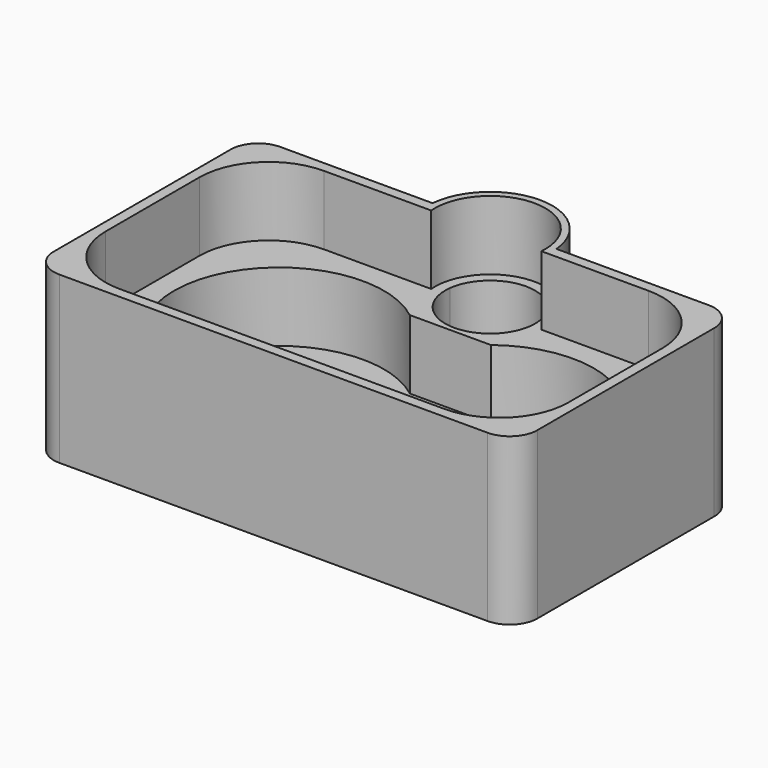
from build123d import *

# Parameters (mm, degrees)
F1_DEPTH = 2
F2_DEPTH = 5
F4_DEPTH = 5
F5_R     = 2
F6_R     = 5


# Not quite as in the source:
# - a feature names something its author has since deleted; it is built from what else it names


with BuildPart() as f1:
    # F0 (on Top) → F1 (new body)
    with BuildSketch(Plane.XY):
        with BuildLine():
            ThreePointArc((4.4821870069, 10), (0, 14.100000456), (-4.4821870069, 10))
            Line((-4.4821870069, 10), (-3.2252907411, 10))
            ThreePointArc((-3.2252907411, 10), (0, 12.850000456), (3.2252907411, 10))
            Line((3.2252907411, 10), (4.4821870069, 10))
        make_face()
        with BuildLine():
            Line((3.2252907411, 10), (-3.2252907411, 10))
            ThreePointArc((-3.2252907411, 10), (-0.2003810013, 6.3561836525), (3.25, 9.600000456))
            ThreePointArc((3.25, 9.600000456), (3.2438168034, 9.8003814573), (3.2252907411, 10))
        make_face()
        with BuildLine():
            ThreePointArc((3.2252907411, 10), (0, 12.850000456), (-3.2252907411, 10))
            Line((-3.2252907411, 10), (3.2252907411, 10))
        make_face()
        with BuildLine():
            ThreePointArc((-2.9352384841, 6), (-0.7731344117, 3.3397464334), (0, 0))
            ThreePointArc((0, 0), (0.7731344117, 3.3397464334), (2.9352384841, 6))
            Line((2.9352384841, 6), (2.699999392, 6))
            ThreePointArc((2.699999392, 6), (0, 5.100000456), (-2.699999392, 6))
            Line((-2.699999392, 6), (-2.9352384841, 6))
        make_face()
        with BuildLine():
            ThreePointArc((2.9352384841, -6), (0.7731344117, -3.3397464334), (0, 0))
            ThreePointArc((0, 0), (-0.7731344117, -3.3397464334), (-2.9352384841, -6))
            Line((-2.9352384841, -6), (2.9352384841, -6))
        make_face()
        with BuildLine():
            ThreePointArc((-4.4821870069, 10), (-4.1104683878, 7.768593993), (-2.699999392, 6))
            Line((-2.699999392, 6), (2.699999392, 6))
            ThreePointArc((2.699999392, 6), (4.0249221896, 7.5875389364), (4.5, 9.600000456))
            ThreePointArc((4.5, 9.600000456), (4.495544546, 9.8001984442), (4.4821870069, 10))
            Line((4.4821870069, 10), (3.2252907411, 10))
            ThreePointArc((3.2252907411, 10), (3.2438168034, 9.8003814573), (3.25, 9.600000456))
            ThreePointArc((3.25, 9.600000456), (-0.2003810013, 6.3561836525), (-3.2252907411, 10))
            Line((-3.2252907411, 10), (-4.4821870069, 10))
        make_face()
        with BuildLine():
            ThreePointArc((-2.9352384841, -6), (-0.7731344117, -3.3397464334), (0, 0))
            ThreePointArc((0, 0), (-0.7731344117, 3.3397464334), (-2.9352384841, 6))
            ThreePointArc((-2.9352384841, 6), (-14.6584577236, 2.8174766307), (-8.3490864524, -7.5629934211))
            ThreePointArc((-8.3490864524, -7.5629934211), (-7.6, -6.85), (-6.8509135476, -7.5629934211))
            ThreePointArc((-6.8509135476, -7.5629934211), (-4.7825233693, -7.0584577236), (-2.9352384841, -6))
        make_face()
        with BuildLine():
            ThreePointArc((2.9352384841, 6), (0.7731344117, 3.3397464334), (0, 0))
            ThreePointArc((0, 0), (0.7731344117, -3.3397464334), (2.9352384841, -6))
            ThreePointArc((2.9352384841, -6), (4.7825233693, -7.0584577236), (6.8509135476, -7.5629934211))
            ThreePointArc((6.8509135476, -7.5629934211), (7.6, -6.85), (8.3490864524, -7.5629934211))
            ThreePointArc((8.3490864524, -7.5629934211), (13.2326306926, -5.1023006067), (15.2, 0))
            ThreePointArc((15.2, 0), (10.9397464334, 6.8268655883), (2.9352384841, 6))
        make_face()
        with BuildLine():
            ThreePointArc((-8.3490864524, -7.5629934211), (-14.6584577236, 2.8174766307), (-2.9352384841, 6))
            Line((-2.9352384841, 6), (-2.699999392, 6))
            ThreePointArc((-2.699999392, 6), (-4.1104683878, 7.768593993), (-4.4821870069, 10))
            Line((-4.4821870069, 10), (-17.5, 10))
            Line((-17.5, 10), (-17.5, -10))
            Line((-17.5, -10), (17.5, -10))
            Line((17.5, -10), (17.5, 10))
            Line((17.5, 10), (4.4821870069, 10))
            ThreePointArc((4.4821870069, 10), (4.495544546, 9.8001984442), (4.5, 9.600000456))
            ThreePointArc((4.5, 9.600000456), (4.0249221896, 7.5875389364), (2.699999392, 6))
            Line((2.699999392, 6), (2.9352384841, 6))
            ThreePointArc((2.9352384841, 6), (10.9397464334, 6.8268655883), (15.2, 0))
            ThreePointArc((15.2, 0), (13.2326306926, -5.1023006067), (8.3490864524, -7.5629934211))
            ThreePointArc((8.3490864524, -7.5629934211), (8.3497715783, -7.5814910734), (8.35, -7.6))
            ThreePointArc((8.35, -7.6), (7.5814910734, -8.3497715783), (6.8509135476, -7.5629934211))
            ThreePointArc((6.8509135476, -7.5629934211), (4.7825233693, -7.0584577236), (2.9352384841, -6))
            Line((2.9352384841, -6), (-2.9352384841, -6))
            ThreePointArc((-2.9352384841, -6), (-4.7825233693, -7.0584577236), (-6.8509135476, -7.5629934211))
            ThreePointArc((-6.8509135476, -7.5629934211), (-6.8502284217, -7.5814910734), (-6.85, -7.6))
            ThreePointArc((-6.85, -7.6), (-7.6185089266, -8.3497715783), (-8.3490864524, -7.5629934211))
        make_face()
        with BuildLine():
            ThreePointArc((-6.8509135476, -7.5629934211), (-7.6, -6.85), (-8.3490864524, -7.5629934211))
            ThreePointArc((-8.3490864524, -7.5629934211), (-7.6, -7.6), (-6.8509135476, -7.5629934211))
        make_face()
        with BuildLine():
            ThreePointArc((-6.8509135476, -7.5629934211), (-7.6, -7.6), (-8.3490864524, -7.5629934211))
            ThreePointArc((-8.3490864524, -7.5629934211), (-7.6185089266, -8.3497715783), (-6.85, -7.6))
            ThreePointArc((-6.85, -7.6), (-6.8502284217, -7.5814910734), (-6.8509135476, -7.5629934211))
        make_face()
        with BuildLine():
            ThreePointArc((8.3490864524, -7.5629934211), (7.6, -6.85), (6.8509135476, -7.5629934211))
            ThreePointArc((6.8509135476, -7.5629934211), (7.6, -7.6), (8.3490864524, -7.5629934211))
        make_face()
        with BuildLine():
            ThreePointArc((8.3490864524, -7.5629934211), (7.6, -7.6), (6.8509135476, -7.5629934211))
            ThreePointArc((6.8509135476, -7.5629934211), (7.5814910734, -8.3497715783), (8.35, -7.6))
            ThreePointArc((8.35, -7.6), (8.3497715783, -7.5814910734), (8.3490864524, -7.5629934211))
        make_face()
        with BuildLine():
            Line((2.699999392, 6), (-2.699999392, 6))
            ThreePointArc((-2.699999392, 6), (0, 5.100000456), (2.699999392, 6))
        make_face()
    extrude(amount=-F1_DEPTH)

    # F0 (on Top) → F2 (join)
    with BuildSketch(Plane.XY):
        with BuildLine():
            ThreePointArc((-8.3490864524, -7.5629934211), (-14.6584577236, 2.8174766307), (-2.9352384841, 6))
            Line((-2.9352384841, 6), (-2.699999392, 6))
            ThreePointArc((-2.699999392, 6), (-4.1104683878, 7.768593993), (-4.4821870069, 10))
            Line((-4.4821870069, 10), (-17.5, 10))
            Line((-17.5, 10), (-17.5, -10))
            Line((-17.5, -10), (17.5, -10))
            Line((17.5, -10), (17.5, 10))
            Line((17.5, 10), (4.4821870069, 10))
            ThreePointArc((4.4821870069, 10), (4.495544546, 9.8001984442), (4.5, 9.600000456))
            ThreePointArc((4.5, 9.600000456), (4.0249221896, 7.5875389364), (2.699999392, 6))
            Line((2.699999392, 6), (2.9352384841, 6))
            ThreePointArc((2.9352384841, 6), (10.9397464334, 6.8268655883), (15.2, 0))
            ThreePointArc((15.2, 0), (13.2326306926, -5.1023006067), (8.3490864524, -7.5629934211))
            ThreePointArc((8.3490864524, -7.5629934211), (8.3497715783, -7.5814910734), (8.35, -7.6))
            ThreePointArc((8.35, -7.6), (7.5814910734, -8.3497715783), (6.8509135476, -7.5629934211))
            ThreePointArc((6.8509135476, -7.5629934211), (4.7825233693, -7.0584577236), (2.9352384841, -6))
            Line((2.9352384841, -6), (-2.9352384841, -6))
            ThreePointArc((-2.9352384841, -6), (-4.7825233693, -7.0584577236), (-6.8509135476, -7.5629934211))
            ThreePointArc((-6.8509135476, -7.5629934211), (-6.8502284217, -7.5814910734), (-6.85, -7.6))
            ThreePointArc((-6.85, -7.6), (-7.6185089266, -8.3497715783), (-8.3490864524, -7.5629934211))
        make_face()
        with BuildLine():
            ThreePointArc((4.4821870069, 10), (0, 14.100000456), (-4.4821870069, 10))
            Line((-4.4821870069, 10), (-3.2252907411, 10))
            ThreePointArc((-3.2252907411, 10), (0, 12.850000456), (3.2252907411, 10))
            Line((3.2252907411, 10), (4.4821870069, 10))
        make_face()
        with BuildLine():
            ThreePointArc((-4.4821870069, 10), (-4.1104683878, 7.768593993), (-2.699999392, 6))
            Line((-2.699999392, 6), (2.699999392, 6))
            ThreePointArc((2.699999392, 6), (4.0249221896, 7.5875389364), (4.5, 9.600000456))
            ThreePointArc((4.5, 9.600000456), (4.495544546, 9.8001984442), (4.4821870069, 10))
            Line((4.4821870069, 10), (3.2252907411, 10))
            ThreePointArc((3.2252907411, 10), (3.2438168034, 9.8003814573), (3.25, 9.600000456))
            ThreePointArc((3.25, 9.600000456), (-0.2003810013, 6.3561836525), (-3.2252907411, 10))
            Line((-3.2252907411, 10), (-4.4821870069, 10))
        make_face()
    extrude(amount=F2_DEPTH)

    # F3 (on face) → F4 (join)
    with BuildSketch(Plane.XY.offset(5)):
        with BuildLine():
            Line((17.5, -10), (17.5, 10))
            Line((17.5, 10), (4.4821870069, 10))
            ThreePointArc((4.4821870069, 10), (0, 14.100000456), (-4.4821870069, 10))
            Line((-4.4821870069, 10), (-17.5, 10))
            Line((-17.5, 10), (-17.5, -10))
            Line((-17.5, -10), (17.5, -10))
        make_face()
        with BuildLine():
            Line((3.9846580381, 9.25), (16.75, 9.25))
            Line((16.75, 9.25), (16.75, -9.25))
            Line((16.75, -9.25), (-16.75, -9.25))
            Line((-16.75, -9.25), (-16.75, 9.25))
            Line((-16.75, 9.25), (-3.9846580381, 9.25))
            ThreePointArc((-3.9846580381, 9.25), (-0.1751682727, 13.5961631249), (4, 9.600000456))
            ThreePointArc((4, 9.600000456), (3.9961626689, 9.4248321833), (3.9846580381, 9.25))
        make_face(mode=Mode.SUBTRACT)
    extrude(amount=F4_DEPTH)

    # F5
    f5_edges = [f1.edges().sort_by_distance(p)[0] for p in [
        (-17.5, 10, 4),
        (17.5, 10, 4),
        (17.5, -10, 4),
        (-17.5, -10, 4),
    ]]
    fillet(f5_edges, radius=F5_R)

    # F6
    f6_edges = [f1.edges().sort_by_distance(p)[0] for p in [
        (16.75, -9.25, 7.5),
        (-16.75, -9.25, 7.5),
        (16.75, 9.25, 7.5),
        (-16.75, 9.25, 7.5),
    ]]
    fillet(f6_edges, radius=F6_R)


solid = f1.part
